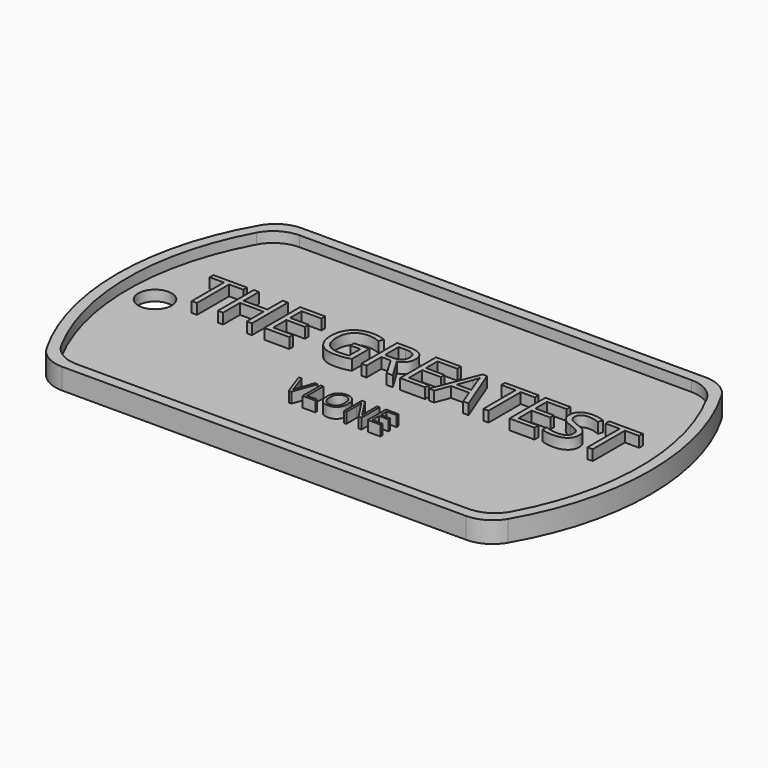
from build123d import *

# Parameters (mm, degrees)
F1_DEPTH       = 1
F3_DEPTH       = 1
F4_R           = 1.5875
F5_DEPTH       = 1
F6_TEXT_SIZE   = 5.9863416633
F6_TEXT_SIZE_2 = 3.0241932513
F7_DEPTH       = 1


# Not quite as in the source:
# - Text() gives the source's letters only with a copy of the font that has no kerning and outlines rounded to 1/6400 em; it was checked with that copy


with BuildPart() as f1:
    # F0 (on Top) → F1 (new body)
    with BuildSketch(Plane.XY):
        with BuildLine():
            ThreePointArc((-19.2474145991, 14.2875), (-20.8349145991, 13.862130657), (-21.9970452561, 12.7))
            ThreePointArc((-21.9970452561, 12.7), (-25.4, 0), (-21.9970452561, -12.7))
            ThreePointArc((-21.9970452561, -12.7), (-20.8349145991, -13.862130657), (-19.2474145991, -14.2875))
            Line((-19.2474145991, -14.2875), (19.2474145991, -14.2875))
            ThreePointArc((19.2474145991, -14.2875), (20.8349145991, -13.862130657), (21.9970452561, -12.7))
            ThreePointArc((21.9970452561, -12.7), (25.4, 0), (21.9970452561, 12.7))
            ThreePointArc((21.9970452561, 12.7), (20.8349145991, 13.862130657), (19.2474145991, 14.2875))
            Line((19.2474145991, 14.2875), (-19.2474145991, 14.2875))
        make_face()
    extrude(amount=F1_DEPTH)

    # F2 (on face) → F3 (join)
    with BuildSketch(Plane.XY.offset(1)):
        with BuildLine():
            Line((19.2474145991, 14.2875), (-19.2474145991, 14.2875))
            ThreePointArc((-19.2474145991, 14.2875), (-20.8349145991, 13.862130657), (-21.9970452561, 12.7))
            ThreePointArc((-21.9970452561, 12.7), (-25.4, 0), (-21.9970452561, -12.7))
            ThreePointArc((-21.9970452561, -12.7), (-20.8349145991, -13.862130657), (-19.2474145991, -14.2875))
            Line((-19.2474145991, -14.2875), (19.2474145991, -14.2875))
            ThreePointArc((19.2474145991, -14.2875), (20.8349145991, -13.862130657), (21.9970452561, -12.7))
            ThreePointArc((21.9970452561, -12.7), (25.4, 0), (21.9970452561, 12.7))
            ThreePointArc((21.9970452561, 12.7), (20.8349145991, 13.862130657), (19.2474145991, 14.2875))
        make_face()
        with BuildLine():
            ThreePointArc((-21.4526124879, 11.6252061249), (-20.2856017842, 12.8404540819), (-18.6611352482, 13.2875))
            Line((-18.6611352482, 13.2875), (18.6611352482, 13.2875))
            ThreePointArc((18.6611352482, 13.2875), (20.2856017842, 12.8404540819), (21.4526124879, 11.6252061249))
            ThreePointArc((21.4526124879, 11.6252061249), (24.4, 0), (21.4526124879, -11.6252061249))
            ThreePointArc((21.4526124879, -11.6252061249), (20.2856017842, -12.8404540819), (18.6611352482, -13.2875))
            Line((18.6611352482, -13.2875), (-18.6611352482, -13.2875))
            ThreePointArc((-18.6611352482, -13.2875), (-20.2856017842, -12.8404540819), (-21.4526124879, -11.6252061249))
            ThreePointArc((-21.4526124879, -11.6252061249), (-24.4, 0), (-21.4526124879, 11.6252061249))
        make_face(mode=Mode.SUBTRACT)
    extrude(amount=F3_DEPTH)

    # F4 (on face) → F5 (cut)
    with BuildSketch(Plane.XY.offset(1)):
        with Locations((-21.821282804, 0)):
            Circle(F4_R)
    extrude(amount=-F5_DEPTH, mode=Mode.SUBTRACT)

    # F6 (on face) → F7 (join)
    with BuildSketch(Plane.XY.offset(1)):
        with Locations((-19.7263992177, 0)):
            Text('THE GREATEST', F6_TEXT_SIZE, font='Open Sans', text_align=(TextAlign.LEFT, TextAlign.BOTTOM))
        with Locations((-4.4271794613, -6.7767836154)):
            Text('VLONE', F6_TEXT_SIZE_2, font='Open Sans', text_align=(TextAlign.LEFT, TextAlign.BOTTOM))
    extrude(amount=F7_DEPTH)


solid = f1.part
